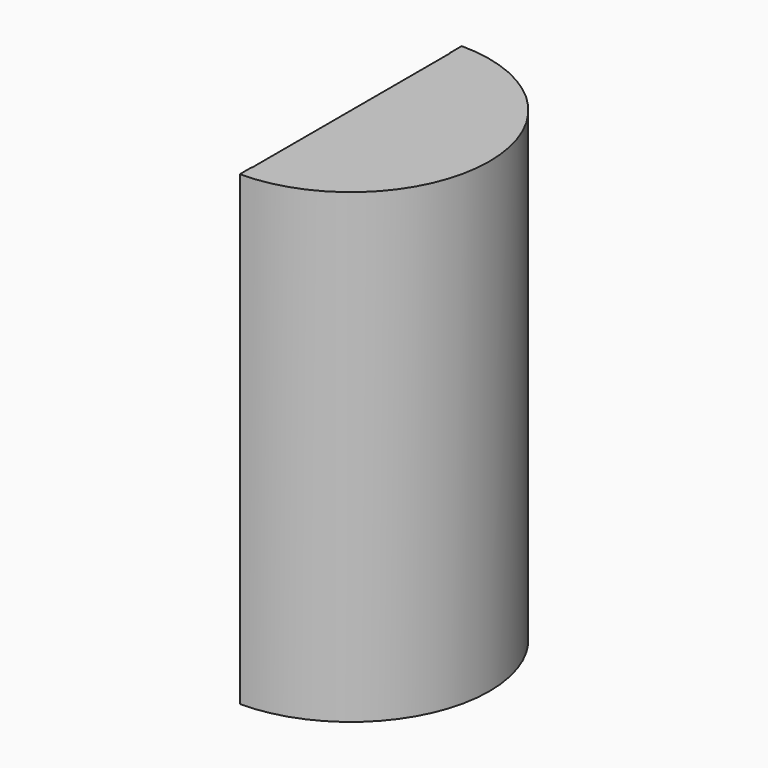
from build123d import *

# Parameters (mm, degrees)
F1_DEPTH    = 19.05
F3_DEPTH    = 0.75946
F4_T4_DEPTH = 76.9415838332
F4_S5_R     = 10.287
F4_T6_DEPTH = 40


# Not quite as in the source:
# - a fillet or chamfer that OpenCascade refuses, or shapes differently, is made with other operations: its cross-section is extruded or revolved along the edge and cut away or added


with BuildPart() as f1:
    # F0 (on Top) → F1 (new body, symmetric)
    with BuildSketch(Plane.XY):
        with BuildLine():
            ThreePointArc((0, 10.287), (10.287, 0), (0, -10.287))
            Line((0, -10.287), (0, -11.557))
            ThreePointArc((0, -11.557), (11.557, 0), (0, 11.557))
            Line((0, 11.557), (0, 10.287))
        make_face()
    extrude(amount=F1_DEPTH, both=True)

    # F2 (on face) → F3 (join, symmetric)
    with BuildSketch(Plane.XY.offset(19.05)):
        with BuildLine():
            Line((0, 11.557), (0, -11.557))
            ThreePointArc((0, -11.557), (11.557, 0), (0, 11.557))
        make_face()
    extrude(amount=F3_DEPTH, both=True)

    # F4: chamfer of 1.524 x 10.8438234569 on 1 edges, made by hand


with BuildPart() as f4_tool2:
    # F4_s3 → F4_t4 (new body)
    with BuildSketch(Plane.XZ.offset(-38.4707919166)):
        Polygon((0, 19.81454), (10.8438234569, 18.29054), (0, 18.29054), align=None)
    extrude(amount=F4_T4_DEPTH)

    # F4_s5 → F4_t6 (intersect, symmetric)
    with BuildSketch(Plane.XY.offset(19.1)):
        Circle(F4_S5_R)
    extrude(amount=F4_T6_DEPTH, both=True, mode=Mode.INTERSECT)


with BuildPart() as f1_1:
    add(f1.part)

    # F4_t1: cut F4_tool2
    add(f4_tool2.part, mode=Mode.SUBTRACT)


solid = f1_1.part
